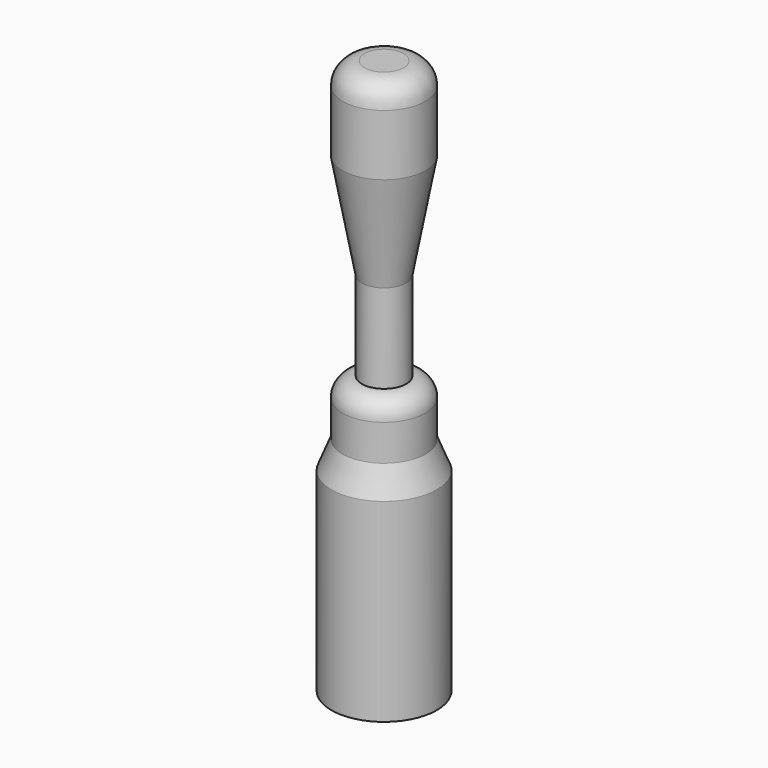
from build123d import *


# Not quite as in the source:
# - ends of sketch curves that miss each other by under 0.0002 mm in the source are joined


with BuildPart() as f1:
    # F0 (on Front) → F1 (revolve)
    with BuildSketch(Plane.XZ):
        with BuildLine():
            Line((3.5, 0), (0, 0))
            Line((0, 0), (0, -100))
            Line((0, -100), (9.5, -100))
            Line((9.5, -100), (9.5, -65))
            Line((9.5, -65), (7.5, -60))
            Line((7.5, -60), (7.5, -53.4999954539))
            ThreePointArc((7.5, -53.4999954539), (6.4748737342, -51.0251217197), (4, -49.9999954539))
            Line((4, -49.9999954539), (4, -34))
            Line((4, -34), (7.5, -15))
            Line((7.5, -15), (7.5, -4))
            ThreePointArc((7.5, -4), (6.3284271247, -1.1715728753), (3.5, 0))
        make_face()
    revolve(axis=Axis((0, 0, -50), (0, 0, 1)))


solid = f1.part
